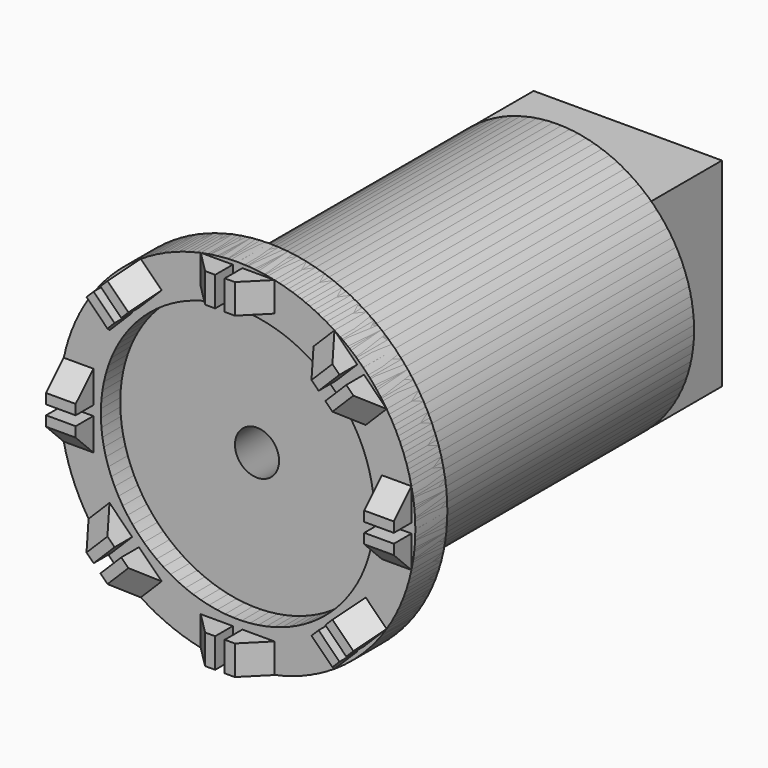
from build123d import *

# Parameters (mm, degrees)
F2_W     = 7.2803417351
F2_H     = 6.7025734382
F3_DEPTH = 5
F4_SIZE  = 4.99999
F5_COUNT = 8
F6_W     = 42.6562729647
F6_H     = 45.0660675903
F6_R     = 5
F7_DEPTH = 20


# Not quite as in the source:
# - a fillet or chamfer is up to 0.001 mm smaller than in the source, because OpenCascade refuses the exact size


with BuildPart() as f1:
    # F0 (on Right) → F1 (revolve)
    with BuildSketch(Plane.YZ):
        Polygon((45.533747226, 5), (55.533747226, 5), (55.533747226, 31.026231125), (-19.466252774, 31.026231125), (-25.8840825409, 40.2705445886), (-34.9619958587, 40.2705445886), (-34.9619958587, 31.026231125), (-29.466252774, 31.026231125), (-29.466252774, 5), (-19.466252774, 5), (-19.466252774, 20), (45.533747226, 20), align=None)
    revolve(axis=Axis((0, -1.2710951269, 0), (0, -1, 0)))

    # F2 (on face) → F3 (join)
    with BuildSketch(Plane.XZ.offset(34.9619958587)):
        with Locations((4.722733709, 36.0413342714)):
            Rectangle(F2_W, F2_H)
        with Locations((-4.722733709, 36.0413342714)):
            Rectangle(F2_W, F2_H)
    extrude(amount=F3_DEPTH)

    # F4 (size 5 in the source; OpenCascade refuses exactly that, so slightly less here)
    f4_edges = [f1.edges().sort_by_distance(p)[0] for p in [
        (-8.362905, -39.961996, 36.041334),
        (8.362905, -39.961996, 36.041334),
    ]]
    chamfer(f4_edges, length=F4_SIZE)


with BuildPart() as f5_1:
    # F5: instance of F1
    add(f1.part.rotate(Axis((0, -1.2710951269, 0), (0, -1, 0)), 1 * 360 / F5_COUNT))


with BuildPart() as f5_2:
    # F5: instance of F1
    add(f1.part.rotate(Axis((0, -1.2710951269, 0), (0, -1, 0)), 2 * 360 / F5_COUNT))


with BuildPart() as f5_3:
    # F5: instance of F1
    add(f1.part.rotate(Axis((0, -1.2710951269, 0), (0, -1, 0)), 3 * 360 / F5_COUNT))


with BuildPart() as f5_4:
    # F5: instance of F1
    add(f1.part.rotate(Axis((0, -1.2710951269, 0), (0, -1, 0)), 4 * 360 / F5_COUNT))


with BuildPart() as f5_5:
    # F5: instance of F1
    add(f1.part.rotate(Axis((0, -1.2710951269, 0), (0, -1, 0)), 5 * 360 / F5_COUNT))


with BuildPart() as f5_6:
    # F5: instance of F1
    add(f1.part.rotate(Axis((0, -1.2710951269, 0), (0, -1, 0)), 6 * 360 / F5_COUNT))


with BuildPart() as f5_7:
    # F5: instance of F1
    add(f1.part.rotate(Axis((0, -1.2710951269, 0), (0, -1, 0)), 7 * 360 / F5_COUNT))


with BuildPart() as f7:
    # F6 (on face) → F7 (new body)
    with BuildSketch(Plane(origin=(0, 55.533747226, 0), x_dir=(-1, 0, 0), z_dir=(0, 1, 0))):
        Rectangle(F6_W, F6_H)
        Circle(F6_R, mode=Mode.SUBTRACT)
    extrude(amount=F7_DEPTH)


solid = Compound([f1.part, f5_1.part, f5_2.part, f5_3.part, f5_4.part, f5_5.part, f5_6.part, f5_7.part, f7.part])
